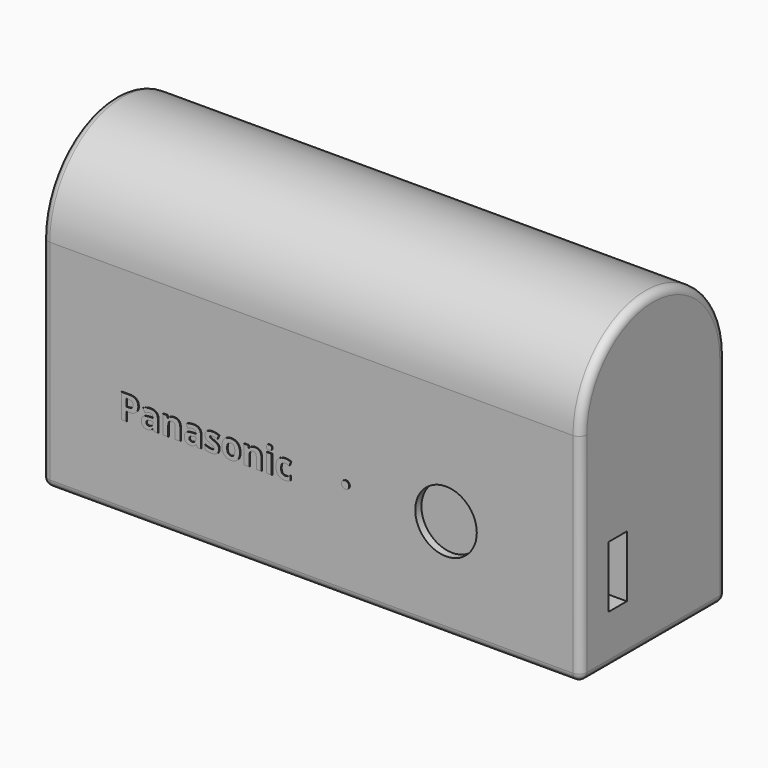
from build123d import *

# Parameters (mm, degrees)
F0_W         = 23.6
F0_H         = 28.2
F1_DEPTH     = 35
F2_TEXT_SIZE = 4.4338643716
F3_DEPTH     = 0.1
F4_R         = 4
F5_DEPTH     = 1
F6_W         = 13.5
F6_H         = 6
F7_DEPTH     = 25
F8_W         = 3
F8_H         = 8
F9_DEPTH     = 10
F10_R        = 1
F11_R        = 0.5
F12_DEPTH    = 0.1


# Not quite as in the source:
# - Text() gives the source's letters only with a copy of the font that has no kerning and outlines rounded to 1/6400 em; it was checked with that copy


with BuildPart() as f1:
    # F0 (on Right) → F1 (new body, symmetric)
    with BuildSketch(Plane.YZ):
        with Locations((0, 14.1)):
            Rectangle(F0_W, F0_H)
        with BuildLine():
            ThreePointArc((11.8, 28.2), (0, 40), (-11.8, 28.2))
            Line((-11.8, 28.2), (11.8, 28.2))
        make_face()
    extrude(amount=F1_DEPTH, both=True)

    # F4 (on face) → F5 (cut)
    with BuildSketch(Plane.XZ.offset(11.8)):
        with Locations((17.5, 13)):
            Circle(F4_R)
    extrude(amount=-F5_DEPTH, mode=Mode.SUBTRACT)

    # F6 (on face) → F7 (cut)
    with BuildSketch(Plane(origin=(-35, 0, 0), x_dir=(0, -1, 0), z_dir=(-1, 0, 0))):
        with Locations((0, 12)):
            Rectangle(F6_W, F6_H)
    extrude(amount=-F7_DEPTH, mode=Mode.SUBTRACT)

    # F8 (on face) → F9 (cut)
    with BuildSketch(Plane.YZ.offset(35)):
        with Locations((-5.8, 10.5)):
            Rectangle(F8_W, F8_H)
    extrude(amount=-F9_DEPTH, mode=Mode.SUBTRACT)

    # F10
    f10_edges = [f1.edges().sort_by_distance(p)[0] for p in [
        (0, -11.8, 0),
        (-35, 0, 0),
        (0, 11.8, 0),
        (35, 0, 0),
        (-35, -11.8, 14.1),
        (-35, 11.8, 14.1),
        (35, -11.8, 14.1),
        (35, 11.8, 14.1),
        (35, 0, 40),
        (-35, 0, 40),
    ]]
    fillet(f10_edges, radius=F10_R)


with BuildPart() as f3:
    # F2 (on face) → F3 (new body)
    with BuildSketch(Plane.XZ.offset(11.8)):
        with Locations((-25, 11)):
            Text('Panasonic', F2_TEXT_SIZE, font='Open Sans', font_style=FontStyle.BOLD, text_align=(TextAlign.LEFT, TextAlign.BOTTOM))
    extrude(amount=F3_DEPTH)


with BuildPart() as f12:
    # F11 (on face) → F12 (new body)
    with BuildSketch(Plane.XZ.offset(11.8)):
        with Locations((4.5, 13)):
            Circle(F11_R)
    extrude(amount=F12_DEPTH)


solid = Compound([f1.part, f3.part, f12.part])
